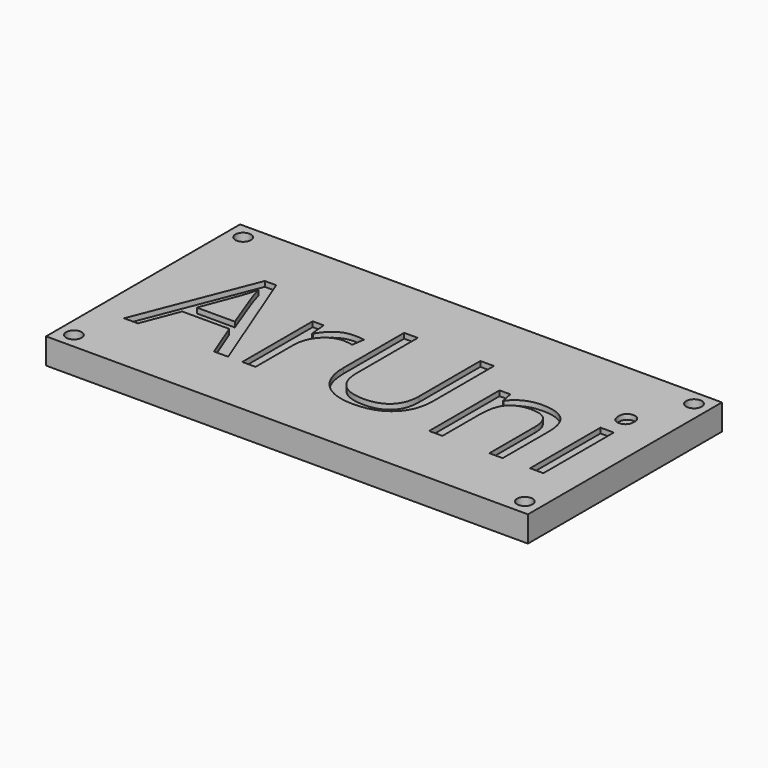
from build123d import *

# Parameters (mm, degrees)
F0_W         = 93.4
F0_H         = 47
F0_R         = 1.5
F1_DEPTH     = 5
F2_TEXT_SIZE = 31.8781377347
F3_DEPTH     = 1


# Not quite as in the source:
# - a feature names something its author has since deleted; it is built from what else it names
# - Text() gives the source's letters only with a copy of the font that has no kerning and outlines rounded to 1/6400 em; it was checked with that copy


with BuildPart() as f1:
    # F0 (on Top) → F1 (new body)
    with BuildSketch(Plane.XY):
        with Locations((-22.9209892631, -9.5544784665)):
            Rectangle(F0_W, F0_H)
        with Locations((-66.6209892631, -30.0544784665)):
            Circle(F0_R, mode=Mode.SUBTRACT)
        with Locations((20.7790107369, -30.0544784665)):
            Circle(F0_R, mode=Mode.SUBTRACT)
        with Locations((-66.6209892631, 10.9455215335)):
            Circle(F0_R, mode=Mode.SUBTRACT)
        with Locations((20.7790107369, 10.9455215335)):
            Circle(F0_R, mode=Mode.SUBTRACT)
    extrude(amount=F1_DEPTH)

    # F2 (on face) → F3 (cut)
    with BuildSketch(Plane.XY.offset(5)):
        with Locations((-64.1047731042, -21.0591931827)):
            Text('ArUni', F2_TEXT_SIZE, font='Open Sans', text_align=(TextAlign.LEFT, TextAlign.BOTTOM))
    extrude(amount=-F3_DEPTH, mode=Mode.SUBTRACT)


solid = f1.part
